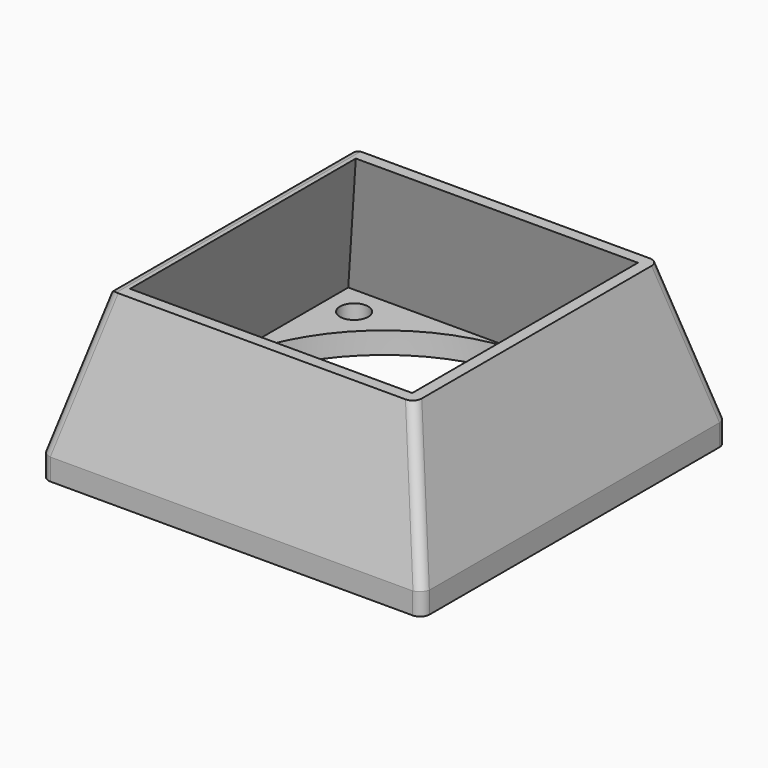
from build123d import *

# Parameters (mm, degrees)
F0_W         = 40.5
F0_H         = 40.5
F2_W         = 32.47
F2_H         = 32.47
F4_W         = 38
F4_H         = 38
F5_W         = 30
F5_H         = 30
F7_W         = 40.5
F7_H         = 40.5
F7_R         = 1.5
F7_R_2       = 19
F8_DEPTH     = 2.3
F9_T3_DEPTH  = 22.3515662211
F9_T6_DEPTH  = 9.05
F9_T9_DEPTH  = 9.05
F9_T12_DEPTH = 22.3515662211
F9_T15_DEPTH = 22.3515662211
F9_T18_DEPTH = 9.05
F9_T21_DEPTH = 22.3515662211
F9_T24_DEPTH = 9.05
F9_T27_DEPTH = 36.3076821333


# Not quite as in the source:
# - a fillet or chamfer that OpenCascade refuses, or shapes differently, is made with other operations: its cross-section is extruded or revolved along the edge and cut away or added


with BuildPart() as f3:
    # F0 (on Top) → F3 section 0
    with BuildSketch(Plane.XY):
        Rectangle(F0_W, F0_H)
    # F2 (on offset) → F3 section 1
    with BuildSketch(Plane.XY.offset(15)):
        Rectangle(F2_W, F2_H)
    loft()

    # F4 (on face) → F6 section 0
    with BuildSketch(Plane.XY):
        Rectangle(F4_W, F4_H)
    # F5 (on face) → F6 section 1
    with BuildSketch(Plane.XY.offset(15)):
        Rectangle(F5_W, F5_H)
    loft(mode=Mode.SUBTRACT)

    # F7 (on face) → F8 (join)
    with BuildSketch(Plane.XY):
        Rectangle(F7_W, F7_H)
        with Locations((-15.9099025767, -15.9099025767)):
            Circle(F7_R, mode=Mode.SUBTRACT)
        with Locations((15.9099025767, -15.9099025767)):
            Circle(F7_R, mode=Mode.SUBTRACT)
        with Locations((-15.9099025767, 15.9099025767)):
            Circle(F7_R, mode=Mode.SUBTRACT)
        Circle(F7_R_2, mode=Mode.SUBTRACT)
        with Locations((15.9099025767, 15.9099025767)):
            Circle(F7_R, mode=Mode.SUBTRACT)
    extrude(amount=-F8_DEPTH)

    # F9: fillet of radius 1 on 9 edges, made by hand


with BuildPart() as f9_tool1:
    # F9_s2 → F9_t3 (new body)
    with BuildSketch(Plane(origin=(-3.5329799901, -3.5329799901, -13.1991780453), x_dir=(-0.7071067812, 0.7071067812, 0), z_dir=(0.2503317407, 0.2503317407, 0.9352368893))):
        with BuildLine():
            ThreePointArc((-0.6830609237, 26.1443262584), (0, 26.4139648585), (0.6830609237, 26.1443262584))
            Line((0.6830609237, 26.1443262584), (0, 26.783150032))
            Line((0, 26.783150032), (-0.6830609237, 26.1443262584))
        make_face()
    extrude(amount=F9_T3_DEPTH)


with BuildPart() as f9_tool4:
    # F9_s5 → F9_t6 (new body)
    with BuildSketch(Plane.XY.offset(4.25)):
        with BuildLine():
            ThreePointArc((-19.25, -20.25), (-19.9571067812, -19.9571067812), (-20.25, -19.25))
            Line((-20.25, -19.25), (-20.25, -20.25))
            Line((-20.25, -20.25), (-19.25, -20.25))
        make_face()
    extrude(amount=-F9_T6_DEPTH)


with BuildPart() as f9_tool7:
    # F9_s8 → F9_t9 (new body)
    with BuildSketch(Plane.XY.offset(4.25)):
        with BuildLine():
            ThreePointArc((-20.25, 19.25), (-19.9571067812, 19.9571067812), (-19.25, 20.25))
            Line((-19.25, 20.25), (-20.25, 20.25))
            Line((-20.25, 20.25), (-20.25, 19.25))
        make_face()
    extrude(amount=-F9_T9_DEPTH)


with BuildPart() as f9_tool10:
    # F9_s11 → F9_t12 (new body)
    with BuildSketch(Plane(origin=(-3.5329799901, 3.5329799901, -13.1991780453), x_dir=(0.7071067812, 0.7071067812, 0), z_dir=(0.2503317407, -0.2503317407, 0.9352368893))):
        with BuildLine():
            ThreePointArc((-0.6830609237, 26.1443262584), (0, 26.4139648585), (0.6830609237, 26.1443262584))
            Line((0.6830609237, 26.1443262584), (0, 26.783150032))
            Line((0, 26.783150032), (-0.6830609237, 26.1443262584))
        make_face()
    extrude(amount=F9_T12_DEPTH)


with BuildPart() as f9_tool13:
    # F9_s14 → F9_t15 (new body)
    with BuildSketch(Plane(origin=(3.5329799901, 3.5329799901, -13.1991780453), x_dir=(0.7071067812, -0.7071067812, 0), z_dir=(-0.2503317407, -0.2503317407, 0.9352368893))):
        with BuildLine():
            ThreePointArc((0.6830609237, 26.1443262584), (0, 26.4139648585), (-0.6830609237, 26.1443262584))
            Line((-0.6830609237, 26.1443262584), (0, 26.783150032))
            Line((0, 26.783150032), (0.6830609237, 26.1443262584))
        make_face()
    extrude(amount=F9_T15_DEPTH)


with BuildPart() as f9_tool16:
    # F9_s17 → F9_t18 (new body)
    with BuildSketch(Plane.XY.offset(4.25)):
        with BuildLine():
            ThreePointArc((20.25, 19.25), (19.9571067812, 19.9571067812), (19.25, 20.25))
            Line((19.25, 20.25), (20.25, 20.25))
            Line((20.25, 20.25), (20.25, 19.25))
        make_face()
    extrude(amount=-F9_T18_DEPTH)


with BuildPart() as f9_tool19:
    # F9_s20 → F9_t21 (new body)
    with BuildSketch(Plane(origin=(3.5329799901, -3.5329799901, -13.1991780453), x_dir=(-0.7071067812, -0.7071067812, 0), z_dir=(-0.2503317407, 0.2503317407, 0.9352368893))):
        with BuildLine():
            ThreePointArc((0.6830609237, 26.1443262584), (0, 26.4139648585), (-0.6830609237, 26.1443262584))
            Line((-0.6830609237, 26.1443262584), (0, 26.783150032))
            Line((0, 26.783150032), (0.6830609237, 26.1443262584))
        make_face()
    extrude(amount=F9_T21_DEPTH)


with BuildPart() as f9_tool22:
    # F9_s23 → F9_t24 (new body)
    with BuildSketch(Plane.XY.offset(4.25)):
        with BuildLine():
            ThreePointArc((19.25, -20.25), (19.9571067812, -19.9571067812), (20.25, -19.25))
            Line((20.25, -19.25), (20.25, -20.25))
            Line((20.25, -20.25), (19.25, -20.25))
        make_face()
    extrude(amount=-F9_T24_DEPTH)


with BuildPart() as f9_tool25:
    # F9_s26 → F9_t27 (new body)
    with BuildSketch(Plane.XZ.offset(-18.1538410667)):
        with BuildLine():
            ThreePointArc((-15.4674635733, 15), (-16.0763295685, 14.7932730929), (-16.4334575956, 14.2585644))
            Line((-16.4334575956, 14.2585644), (-16.235, 15))
            Line((-16.235, 15), (-15.4674635733, 15))
        make_face()
    extrude(amount=F9_T27_DEPTH)


with BuildPart() as f3_1:
    add(f3.part)

    # F9_t28: cut F9_tool1, F9_tool4, F9_tool7, F9_tool10, F9_tool13, F9_tool16, F9_tool19, F9_tool22, F9_tool25
    add([f9_tool1.part, f9_tool4.part, f9_tool7.part, f9_tool10.part, f9_tool13.part, f9_tool16.part, f9_tool19.part, f9_tool22.part, f9_tool25.part], mode=Mode.SUBTRACT)


solid = f3_1.part
